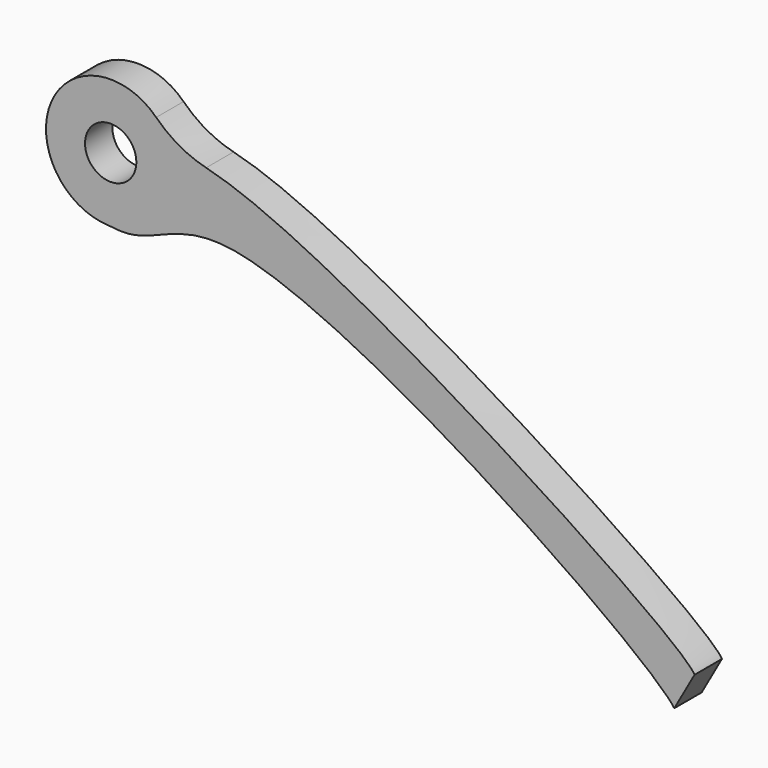
from build123d import *

# Parameters (mm, degrees)
F1_DEPTH = 3.175
F2_R     = 10
F3_R     = 5


# Not quite as in the source:
# - a length typed as a fraction of an inch, garbled in the dataset ("3 / 203.2 mm" for 3/8 in), is restored


with BuildPart() as f1:
    # F0 (on Front) → F1 (new body)
    with BuildSketch(Plane.XZ):
        with BuildLine():
            ThreePointArc((6, 0), (5.9004938384, 1.0881968861), (5.6052758457, 2.1402996738))
            ThreePointArc((5.6052758457, 2.1402996738), (-4.9417506029, 3.4028078081), (0, -6))
            ThreePointArc((0, -6), (4.2426406871, -4.2426406871), (6, 0))
        make_face()
        with BuildLine():
            ThreePointArc((1.9156814293, 1.4143960633), (2.2618651558, 0.7445250698), (2.38125, 0))
            ThreePointArc((2.38125, 0), (-2.2618651558, -0.7445250698), (1.9156814293, 1.4143960633))
        make_face(mode=Mode.SUBTRACT)
        with BuildLine():
            add(Edge.make_bspline(
                [(5.6052758457, 2.1402996738), (8.4837125149, 2.063977977), (22.7725665876, -2.7548580827), (53.0235731676, -22.747897807), (54.1747063398, -25.0206626952)],
                knots=[0.1702278507, 0.1702278507, 0.1702278507, 0.1702278507, 0.381786854, 1, 1, 1, 1], degree=3))
            ThreePointArc((5.6052758457, 2.1402996738), (5.9004938384, 1.0881968861), (6, 0))
            ThreePointArc((6, 0), (4.2426406871, -4.2426406871), (0, -6))
            add(Edge.make_bspline(
                [(0, -6), (3.8225116527, -6.7277911583), (9.1618873845, 3.4044193042), (49.9044501281, -24.856960065), (52.2936917841, -28.3679403365)],
                knots=[0, 0, 0, 0, 0.3265101528, 1, 1, 1, 1], degree=3))
            Line((52.2936917841, -28.3679403365), (54.1747063398, -25.0206626952))
        make_face()
    extrude(amount=F1_DEPTH)

    # F2
    f2_edges = [f1.edges().sort_by_distance(p)[0] for p in [
        (5.605276, -1.5875, 2.1403),
    ]]
    fillet(f2_edges, radius=F2_R)

    # F3
    f3_edges = [f1.edges().sort_by_distance(p)[0] for p in [
        (0, -1.5875, -6),
    ]]
    fillet(f3_edges, radius=F3_R)


solid = f1.part
